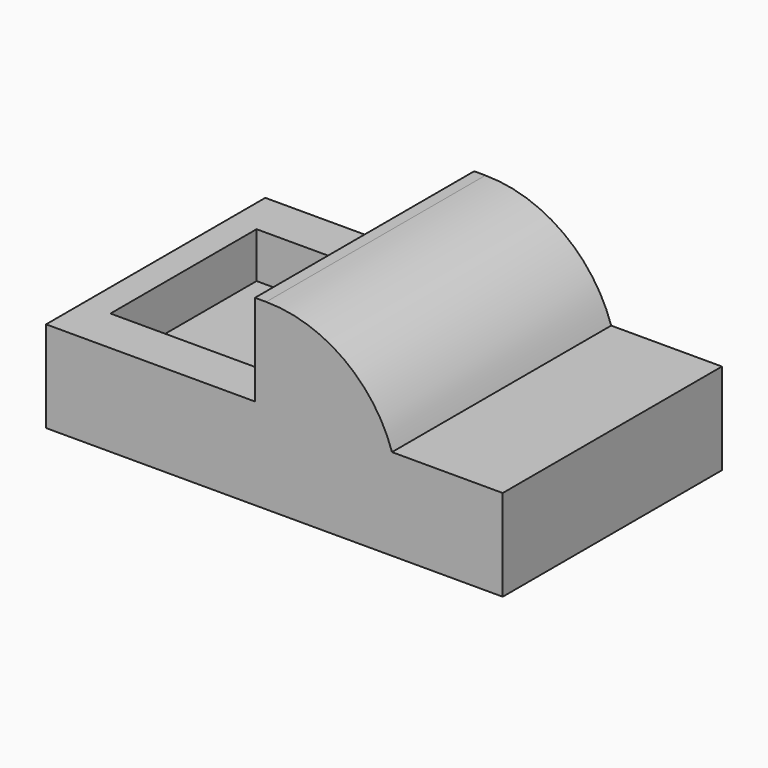
from build123d import *

# Parameters (mm, degrees)
F0_W        = 127
F0_H        = 76.2
F1_DEPTH    = 25.4
F2_W        = 38.1
F2_H        = 76.2
F3_DEPTH    = 25.4
F4_T1_DEPTH = 251.1217558139
F6_DEPTH    = 12.7


# Not quite as in the source:
# - a fillet or chamfer that OpenCascade refuses, or shapes differently, is made with other operations: its cross-section is extruded or revolved along the edge and cut away or added


with BuildPart() as f1:
    # F0 (on Top) → F1 (new body)
    with BuildSketch(Plane.XY):
        with Locations((-4.94965637, -2.3779198527)):
            Rectangle(F0_W, F0_H)
    extrude(amount=F1_DEPTH)

    # F2 (on face) → F3 (join)
    with BuildSketch(Plane.XY.offset(25.4)):
        with Locations((8.6990555257, -2.3779198527)):
            Rectangle(F2_W, F2_H)
    extrude(amount=F3_DEPTH)

    # F4: fillet of radius 36.7926146906 on 1 edges, made by hand

    # F4_s2 → F4_t1 (cut)
    with BuildSketch(Plane.XZ.offset(-123.1829580542)):
        with BuildLine():
            ThreePointArc((27.7490555257, 25.4), (14.3810455558, 43.7803644885), (-7.2352956371, 50.8))
            Line((-7.2352956371, 50.8), (27.7490555257, 50.8))
            Line((27.7490555257, 50.8), (27.7490555257, 25.4))
        make_face()
    extrude(amount=F4_T1_DEPTH, mode=Mode.SUBTRACT)

    # F5 (on face) → F6 (cut)
    with BuildSketch(Plane.XY.offset(25.4)):
        Polygon((-39.4003004222, 23.0220801473), (-60.7068873942, 23.0220801473), (-60.7068873942, -27.7779198527), (-39.4003004222, -27.7779198527), (-17.6245812327, -27.7779198527), (-17.6245812327, 23.0220801473), align=None)
    extrude(amount=-F6_DEPTH, mode=Mode.SUBTRACT)


solid = f1.part
